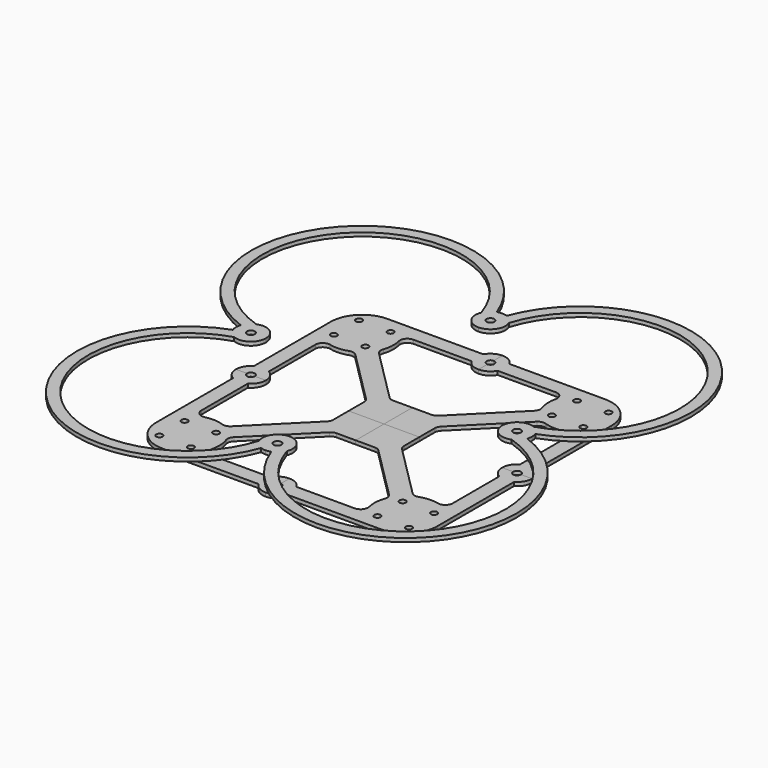
from build123d import *
from build123d import SkipClean  # not in build123d's __all__

# Parameters (mm, degrees)
F1_R     = 0.85
F2_DEPTH = 1
F3_R     = 2
F7_DEPTH = 1


with BuildPart() as f2:
    # F1 (on Top) → F2 (new body)
    with BuildSketch(Plane.XY):
        with BuildLine():
            ThreePointArc((33.9228082029, 22.211705652), (36.8558425766, 25.2997025773), (37.9228082029, 29.4228082029))
            ThreePointArc((37.9228082029, 29.4228082029), (35.433215843, 35.433215843), (29.4228082029, 37.9228082029))
            ThreePointArc((29.4228082029, 37.9228082029), (25.2997025773, 36.8558425766), (22.211705652, 33.9228082029))
            ThreePointArc((22.211705652, 33.9228082029), (20.928169901, 29.7246692972), (21.9104786034, 25.4460125093))
            ThreePointArc((21.9104786034, 25.4460125093), (23.4124005628, 23.4124005628), (25.4460125093, 21.9104786034))
            ThreePointArc((25.4460125093, 21.9104786034), (29.7246692972, 20.928169901), (33.9228082029, 22.211705652))
        make_face()
        with Locations((25.1728082029, 25.1728082029)):
            Circle(F1_R, mode=Mode.SUBTRACT)
        with Locations((33.6728082029, 25.1728082029)):
            Circle(F1_R, mode=Mode.SUBTRACT)
        with Locations((25.1728082029, 33.6728082029)):
            Circle(F1_R, mode=Mode.SUBTRACT)
        with Locations((33.6728082029, 33.6728082029)):
            Circle(F1_R, mode=Mode.SUBTRACT)
        with BuildLine():
            Line((37.9228082029, 3.5217183306), (37.9228082029, 29.4228082029))
            ThreePointArc((37.9228082029, 29.4228082029), (36.8558425766, 25.2997025773), (33.9228082029, 22.211705652))
            Line((33.9228082029, 22.211705652), (33.9228082029, 3.5217183306))
            ThreePointArc((33.9228082029, 3.5217183306), (35.9228082029, 4.05), (37.9228082029, 3.5217183306))
        make_face()
        with BuildLine():
            ThreePointArc((22.211705652, 33.9228082029), (25.2997025773, 36.8558425766), (29.4228082029, 37.9228082029))
            Line((29.4228082029, 37.9228082029), (3.5217183306, 37.9228082029))
            ThreePointArc((3.5217183306, 37.9228082029), (4.05, 35.9228082029), (3.5217183306, 33.9228082029))
            Line((3.5217183306, 33.9228082029), (22.211705652, 33.9228082029))
        make_face()
        with BuildLine():
            ThreePointArc((39.9728082029, 0), (39.4229867698, 2.0374616561), (37.9228082029, 3.5217183306))
            ThreePointArc((37.9228082029, 3.5217183306), (35.9228082029, 4.05), (33.9228082029, 3.5217183306))
            ThreePointArc((33.9228082029, 3.5217183306), (32.422629636, 2.0374616561), (31.8728082029, 0))
            Line((31.8728082029, 0), (34.8728082029, 0))
            ThreePointArc((34.8728082029, 0), (35.9228082029, 1.05), (36.9728082029, 0))
            Line((36.9728082029, 0), (39.9728082029, 0))
        make_face()
        with BuildLine():
            ThreePointArc((3.5217183306, 33.9228082029), (4.05, 35.9228082029), (3.5217183306, 37.9228082029))
            ThreePointArc((3.5217183306, 37.9228082029), (2.0374616561, 39.4229867698), (0, 39.9728082029))
            Line((0, 39.9728082029), (0, 36.9728082029))
            ThreePointArc((0, 36.9728082029), (1.05, 35.9228082029), (0, 34.8728082029))
            Line((0, 34.8728082029), (0, 31.8728082029))
            ThreePointArc((0, 31.8728082029), (2.0374616561, 32.422629636), (3.5217183306, 33.9228082029))
        make_face()
        with BuildLine():
            Line((9.5492883614, 6.0137544555), (25.4460125093, 21.9104786034))
            ThreePointArc((25.4460125093, 21.9104786034), (23.4124005628, 23.4124005628), (21.9104786034, 25.4460125093))
            Line((21.9104786034, 25.4460125093), (6.0137544555, 9.5492883614))
            Line((6.0137544555, 9.5492883614), (0, 9.5492883614))
            Line((0, 9.5492883614), (0, 0))
            Line((0, 0), (9.5492883614, 0))
            Line((9.5492883614, 0), (9.5492883614, 6.0137544555))
        make_face()
    extrude(amount=F2_DEPTH)

    # F3
    f3_edges = [f2.edges().sort_by_distance(p)[0] for p in [
        (33.922808, 22.211706, 0.5),
        (25.446013, 21.910479, 0.5),
        (9.549288, 6.013754, 0.5),
        (6.013754, 9.549288, 0.5),
        (21.910479, 25.446013, 0.5),
        (22.211706, 33.922808, 0.5),
    ]]
    fillet(f3_edges, radius=F3_R)

    # F4: F2 across face


with BuildPart() as f2_1:
    add(f2.part, clean=False)
    with SkipClean():  # cleaning this boolean's faces spoils the solid; the shape is the same uncleaned
        add(f2.part.mirror(Plane(origin=(0, 4.7746441807, 0.5), x_dir=(0, -1, 0), z_dir=(-1, 0, 0))), clean=False)

    # F5: F2 across face


with BuildPart() as f2_2:
    add(f2_1.part, clean=False)
    with SkipClean():  # cleaning this boolean's faces spoils the solid; the shape is the same uncleaned
        add(f2_1.part.mirror(Plane(origin=(4.7746441807, 0, 0.5), x_dir=(1, 0, 0), z_dir=(0, -1, 0))), clean=False)


with BuildPart() as f7:
    # F6 (on Top) → F7 (new body)
    with BuildSketch(Plane.XY):
        with BuildLine():
            ThreePointArc((3.7495508007, 37.4536147853), (48.4439806168, 48.4439806168), (37.4536147853, 3.7495508007))
            ThreePointArc((37.4536147853, 3.7495508007), (38.8510478665, 2.7978406803), (39.7381573955, 1.3585324945))
            ThreePointArc((39.7381573955, 1.3585324945), (50.5653009604, 50.5653009604), (1.3585324945, 39.7381573955))
            ThreePointArc((1.3585324945, 39.7381573955), (2.7978406803, 38.8510478665), (3.7495508007, 37.4536147853))
        make_face()
        with BuildLine():
            ThreePointArc((39.7381573955, 1.3585324945), (38.8510478665, 2.7978406803), (37.4536147853, 3.7495508007))
            ThreePointArc((37.4536147853, 3.7495508007), (33.6641876791, 3.3617158311), (31.8728082029, 0))
            Line((31.8728082029, 0), (34.8728082029, 0))
            ThreePointArc((34.8728082029, 0), (35.9228082029, 1.05), (36.9728082029, 0))
            Line((36.9728082029, 0), (39.9728082029, 0))
            ThreePointArc((39.9728082029, 0), (39.9137143801, 0.6893242234), (39.7381573955, 1.3585324945))
        make_face()
        with BuildLine():
            ThreePointArc((0, 31.8728082029), (3.3617158311, 33.6641876791), (3.7495508007, 37.4536147853))
            ThreePointArc((3.7495508007, 37.4536147853), (2.7978406803, 38.8510478665), (1.3585324945, 39.7381573955))
            ThreePointArc((1.3585324945, 39.7381573955), (0.6893242234, 39.9137143801), (0, 39.9728082029))
            Line((0, 39.9728082029), (0, 36.9728082029))
            ThreePointArc((0, 36.9728082029), (1.05, 35.9228082029), (0, 34.8728082029))
            Line((0, 34.8728082029), (0, 31.8728082029))
        make_face()
    extrude(amount=F7_DEPTH)


with BuildPart() as f7_1:
    # F8: moved
    add(f7.part.moved(Location((0, 0, 10))), clean=False)

    # F9: F7 across plane


with BuildPart() as f7_2:
    add(f7_1.part, clean=False)
    add(f7_1.part.mirror(Plane.YZ), clean=False)

    # F10: F7 across plane


with BuildPart() as f7_3:
    add(f7_2.part, clean=False)
    add(f7_2.part.mirror(Plane.XZ), clean=False)


solid = Compound([f2_2.part, f7_3.part])
